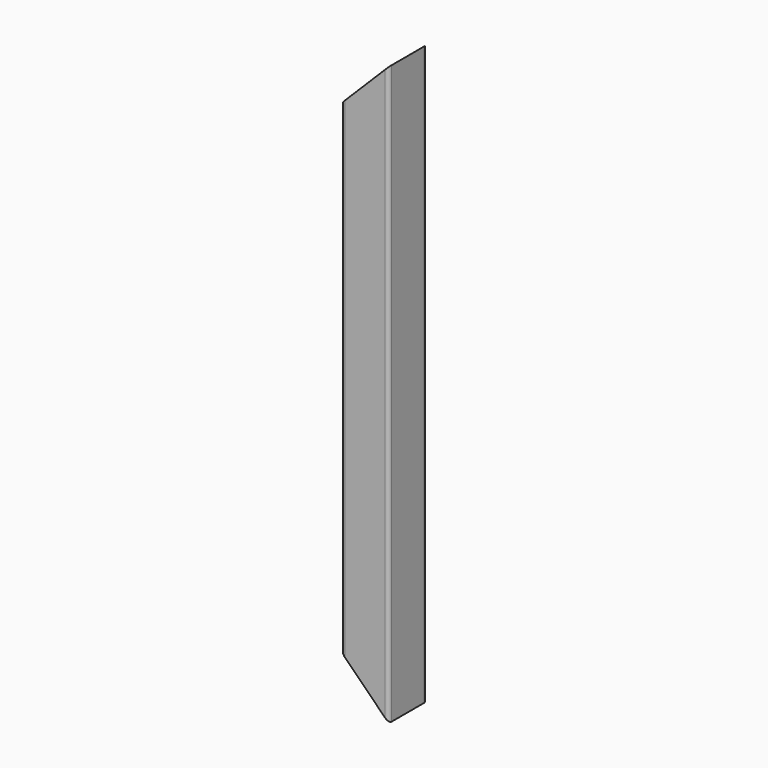
from build123d import *

# Parameters (mm, degrees)
F1_DEPTH      = 243
F3_DEPTH      = 20.001
F3_DEPTH_BACK = 20.001


# Not quite as in the source:
# - a pattern or mirror of a feature is missing from the dataset's text; its kind, count and spacing are read off the source's solid


with BuildPart() as f1:
    # F0 (on Top) → F1 (new body, symmetric)
    with BuildSketch(Plane.XY):
        with BuildLine():
            Line((17, 20), (-17, 20))
            ThreePointArc((-17, 20), (-19.1213203436, 19.1213203436), (-20, 17))
            Line((-20, 17), (-20, -17))
            ThreePointArc((-20, -17), (-19.1213203436, -19.1213203436), (-17, -20))
            Line((-17, -20), (17, -20))
            ThreePointArc((17, -20), (19.1213203436, -19.1213203436), (20, -17))
            Line((20, -17), (20, 17))
            ThreePointArc((20, 17), (19.1213203436, 19.1213203436), (17, 20))
        make_face()
        with BuildLine():
            ThreePointArc((-18, 17), (-17.7071067812, 17.7071067812), (-17, 18))
            Line((-17, 18), (17, 18))
            ThreePointArc((17, 18), (17.7071067812, 17.7071067812), (18, 17))
            Line((18, 17), (18, -17))
            ThreePointArc((18, -17), (17.7071067812, -17.7071067812), (17, -18))
            Line((17, -18), (-17, -18))
            ThreePointArc((-17, -18), (-17.7071067812, -17.7071067812), (-18, -17))
            Line((-18, -17), (-18, 17))
        make_face(mode=Mode.SUBTRACT)
    extrude(amount=F1_DEPTH, both=True)

    # F2 (on Front) → F3 (cut, two sides)
    with BuildSketch(Plane.XZ) as f3_sk:
        Polygon((20, 243), (-20, 243), (-20, 203), align=None)
    f3 = extrude(amount=-F3_DEPTH, mode=Mode.SUBTRACT) + extrude(f3_sk.sketch, amount=F3_DEPTH_BACK, mode=Mode.SUBTRACT)

    # F3_copies: F3 across plane
    add(f3.mirror(Plane(origin=(0, 0, 0), x_dir=(-1, 0, 0), z_dir=(0, 0, -1))), mode=Mode.SUBTRACT)


solid = f1.part
